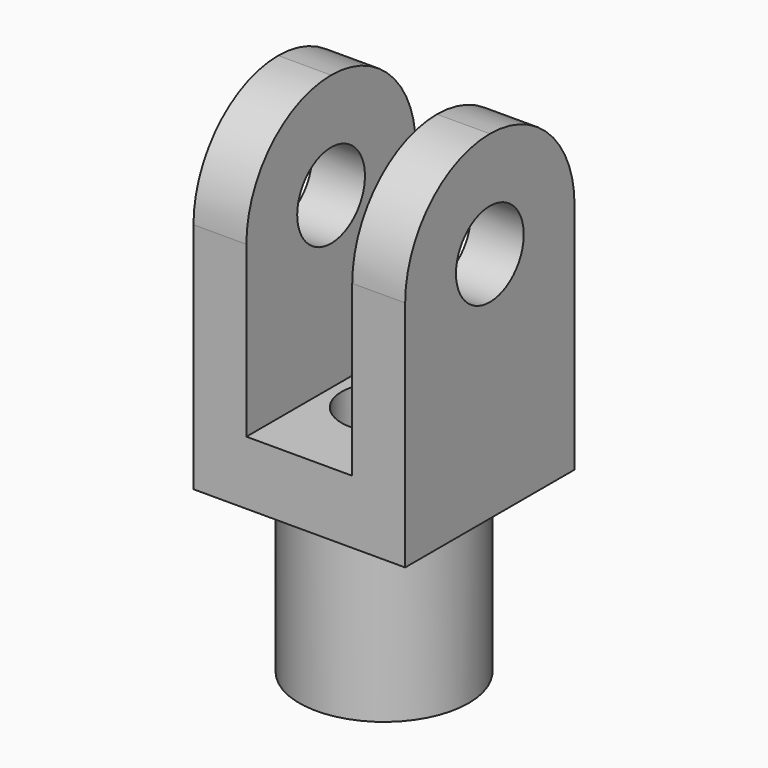
from build123d import *

# Parameters (mm, degrees)
F1_DEPTH = 50
F2_R     = 20
F3_DEPTH = 40
F5_D     = 20
F6_R     = 24.99999
F8_D     = 20
F8_DEPTH = 40.001
F10_D    = 20


# Not quite as in the source:
# - a fillet or chamfer is up to 0.001 mm smaller than in the source, because OpenCascade refuses the exact size


with BuildPart() as f1:
    # F0 (on Front) → F1 (new body)
    with BuildSketch(Plane.XZ):
        Polygon((-25, 80), (-25, 0), (25, 0), (25, 80), (12.5, 80), (12.5, 15), (0, 15), (-12.5, 15), (-12.5, 80), align=None)
    extrude(amount=F1_DEPTH)

    # F2 (on face) → F3 (join)
    with BuildSketch(Plane(origin=(0, 0, 0), x_dir=(1, 0, 0), z_dir=(0, 0, -1))):
        with Locations((0, 25)):
            Circle(F2_R)
    extrude(amount=F3_DEPTH)

    # F5 (through all)
    with Locations(Plane.YZ.offset(25)):
        with Locations((-25, 55)):
            Hole(F5_D / 2)

    # F6 (radius 25 in the source; OpenCascade refuses exactly that, so slightly less here)
    f6_edges = [f1.edges().sort_by_distance(p)[0] for p in [
        (18.75, -50, 80),
        (18.75, 0, 80),
        (-18.75, -50, 80),
        (-18.75, 0, 80),
    ]]
    fillet(f6_edges, radius=F6_R)

    # F8 (through all, one way)
    with BuildSketch(Plane.XY):
        with Locations((0, -25)):
            Circle(F8_D / 2)
    extrude(amount=-F8_DEPTH, mode=Mode.SUBTRACT)

    # F10 (through all)
    with Locations(Plane.XY.offset(15)):
        with Locations((0, -25)):
            Hole(F10_D / 2)


solid = f1.part
